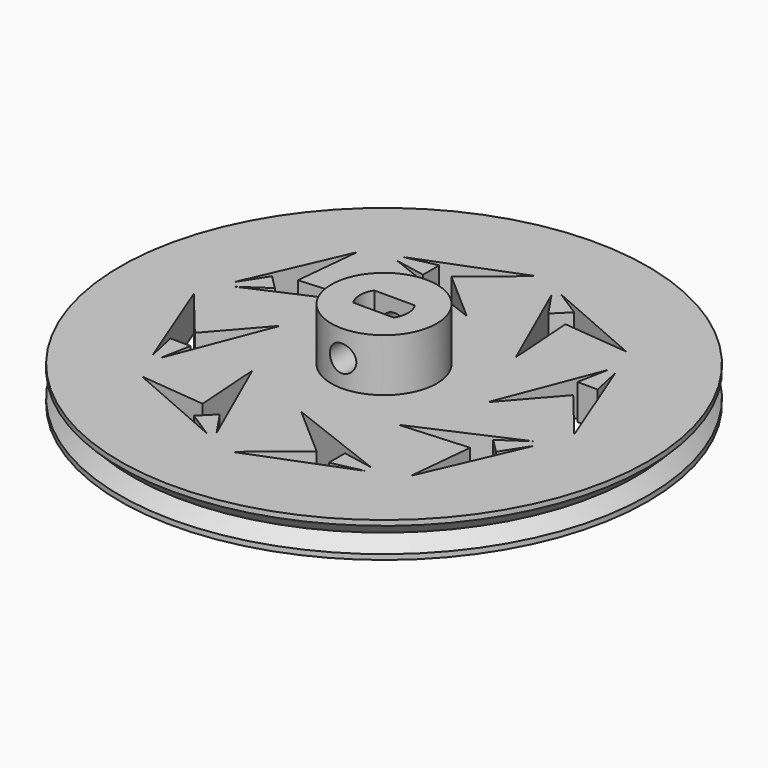
from build123d import *

# Parameters (mm, degrees)
F0_R             = 30
F0_R_2           = 6
F1_DEPTH         = 4
F2_DEPTH         = 6
F3_R             = 1.5
F4_DEPTH         = 7.5
F5_W             = 4.6
F5_H             = 3
F6_DEPTH         = 9.4
F10_DEPTH        = 4
F10_COPIES_COUNT = 8


# Not quite as in the source:
# - a pattern or mirror of a feature is missing from the dataset's text; its kind, count and spacing are read off the source's solid


with BuildPart() as f1:
    # F0 (on Top) → F1 (new body)
    with BuildSketch(Plane.XY):
        Circle(F0_R)
        Circle(F0_R_2, mode=Mode.SUBTRACT)
        Circle(F0_R_2)
    extrude(amount=-F1_DEPTH)

    # F7 (on Front) → F8 (revolve, cut)
    with BuildSketch(Plane.XZ):
        Polygon((-28.5857864376, -2), (-30, -0.5857864376), (-30, -3.4142135624), align=None)
    revolve(axis=Axis((0, 0, 5.5037373677), (0, 0, -1)), mode=Mode.SUBTRACT)

    # F9 (on face) → F10 (cut, through all)
    with BuildSketch(Plane.XY):
        Polygon((-5.8188787661, 16.8492398092), (0, 21.6240715235), (-11.5014315608, 17.1112040934), (-8.0188345164, 17.8686082363), (-8.0188345164, 15.5638335273), (-11.5196653077, 16.2319106039), (0, 11.7657924248), align=None)
    f10 = extrude(amount=-F10_DEPTH, mode=Mode.SUBTRACT)

    # F10_copies: F10 ×8 about axis
    f10_copies_axis = Axis((0, 0, 0), (0, 0, 1))
    for i in range(1, F10_COPIES_COUNT):
        add(f10.rotate(f10_copies_axis, i * 360 / F10_COPIES_COUNT), mode=Mode.SUBTRACT)


with BuildPart() as f2:
    # F0 (on Top) → F2 (new body)
    with BuildSketch(Plane.XY):
        Circle(F0_R_2)
    extrude(amount=F2_DEPTH)

    # F3 (on Front) → F4 (cut, symmetric)
    with BuildSketch(Plane.XZ):
        with Locations((0, 3)):
            Circle(F3_R)
    extrude(amount=F4_DEPTH, both=True, mode=Mode.SUBTRACT)

    # F5 (on face) → F6 (cut)
    with BuildSketch(Plane.XY.offset(6)):
        Rectangle(F5_W, F5_H)
        with BuildLine():
            Line((2.3, 1.5), (2.3, -1.5))
            ThreePointArc((2.3, -1.5), (2.7459060435, 0), (2.3, 1.5))
        make_face()
        with BuildLine():
            ThreePointArc((-2.3, 1.5), (-2.7540939565, 0), (-2.3, -1.5))
            Line((-2.3, -1.5), (-2.3, 1.5))
        make_face()
    extrude(amount=-F6_DEPTH, mode=Mode.SUBTRACT)


solid = Compound([f1.part, f2.part])
